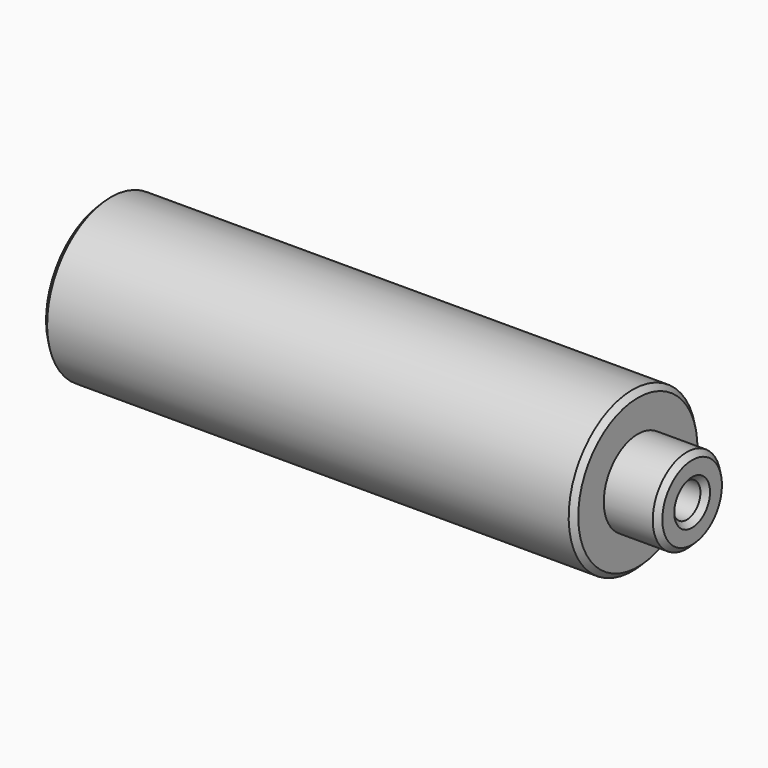
from build123d import *

# Parameters (mm, degrees)
F3_D     = 3.2
F3_DEPTH = 10
F3_TIP   = 0.9613769904
F4_SIZE  = 0.5


with BuildPart() as f1:
    # F0 (on Front) → F1 (revolve)
    with BuildSketch(Plane.XZ):
        Polygon((0, 7.5), (0, 0), (50, 0), (55.1, 0), (55.1, 4), (50, 4), (50, 7.5), align=None)
    revolve(axis=Axis((25, 0, 0), (1, 0, 0)))

    # F3
    with Locations(Plane.YZ.offset(55.1)):
        with Locations((0, 0)):
            Hole(F3_D / 2, depth=F3_DEPTH)
            with Locations((0, 0, -(F3_DEPTH + F3_TIP / 2))):  # 118° drill point
                Cone(0, F3_D / 2, F3_TIP, mode=Mode.SUBTRACT)

    # F4
    f4_edges = [f1.edges().sort_by_distance(p)[0] for p in [
        (50, 0, -7.5),
        (0, 0, -7.5),
        (25, 0, 7.5),
        (55.1, 0, -4),
        (55.1, -1.6, 0),
    ]]
    chamfer(f4_edges, length=F4_SIZE)


solid = f1.part
